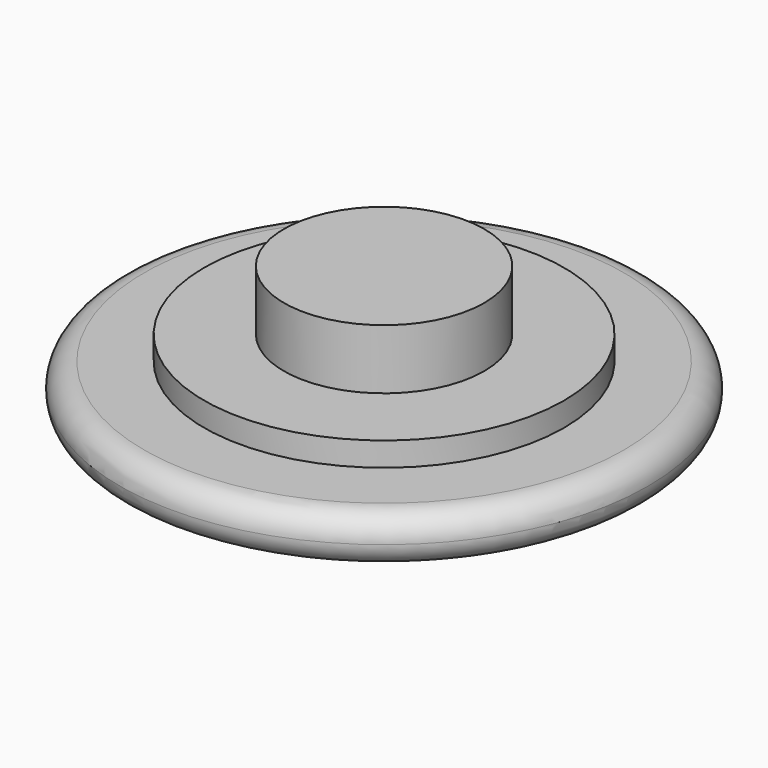
from build123d import *

# Parameters (mm, degrees)
F0_R     = 11
F0_R_2   = 7.5
F1_DEPTH = 2
F0_R_3   = 4.175
F2_DEPTH = 3
F3_DEPTH = 5.5
F4_R     = 0.99999


# Not quite as in the source:
# - a fillet or chamfer is up to 0.001 mm smaller than in the source, because OpenCascade refuses the exact size


with BuildPart() as f1:
    # F0 (on Top) → F1 (new body)
    with BuildSketch(Plane.XY):
        Circle(F0_R)
        Circle(F0_R_2, mode=Mode.SUBTRACT)
    extrude(amount=F1_DEPTH)

    # F0 (on Top) → F2 (join)
    with BuildSketch(Plane.XY):
        Circle(F0_R_2)
        Circle(F0_R_3, mode=Mode.SUBTRACT)
    extrude(amount=F2_DEPTH)

    # F0 (on Top) → F3 (join)
    with BuildSketch(Plane.XY):
        Circle(F0_R_3)
    extrude(amount=F3_DEPTH)

    # F4 (radius 1 in the source; OpenCascade refuses exactly that, so slightly less here)
    f4_edges = [f1.edges().sort_by_distance(p)[0] for p in [
        (-11, 0, 2),
        (-11, 0, 0),
    ]]
    fillet(f4_edges, radius=F4_R)


solid = f1.part
